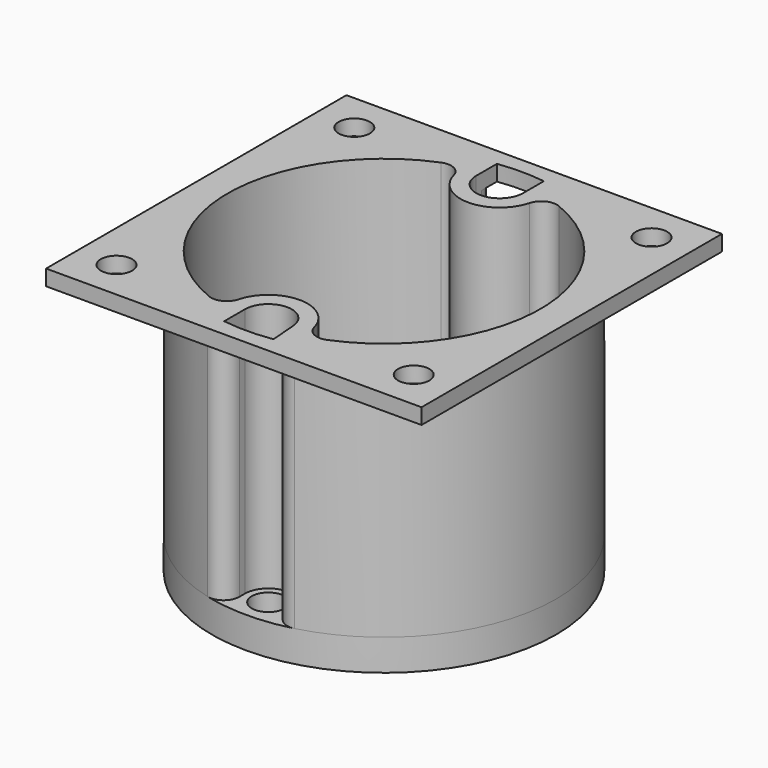
from build123d import *

# Parameters (mm, degrees)
F0_R         = 34.925
F1_DEPTH     = 6.35
F3_DEPTH     = 50.8
F4_R         = 3.3655
F5_DEPTH     = 6.35
F6_W         = 76.2
F6_H         = 76.2
F6_R         = 34.925
F7_DEPTH     = 3.175
F8_R         = 3.175
F9_DEPTH     = 3.175
F10_T1_DEPTH = 50.8
F10_T3_DEPTH = 47.625
F12_DEPTH    = 6.35
F13_R        = 3.175


# Not quite as in the source:
# - a fillet or chamfer that OpenCascade refuses, or shapes differently, is made with other operations: its cross-section is extruded or revolved along the edge and cut away or added


with BuildPart() as f1:
    # F0 (on Top) → F1 (new body)
    with BuildSketch(Plane.XY):
        Circle(F0_R)
    extrude(amount=F1_DEPTH)

    # F2 (on face) → F3 (join)
    with BuildSketch(Plane.XY.offset(6.35)):
        with BuildLine():
            ThreePointArc((4.7625, 29.337), (0, 24.5745), (-4.7625, 29.337))
            Line((-4.7625, 29.337), (-4.7625, 34.5987603644))
            ThreePointArc((-4.7625, 34.5987603644), (-34.925, 0), (-4.7625, -34.5987603644))
            Line((-4.7625, -34.5987603644), (-4.7625, -29.337))
            ThreePointArc((-4.7625, -29.337), (-0.1934429178, -24.5784302477), (4.7467854961, -28.9504334416))
            Line((4.7467854961, -28.9504334416), (5.2016172982, -34.5354716557))
            ThreePointArc((5.2016172982, -34.5354716557), (26.4709473682, -22.7825496912), (34.925, 0))
            ThreePointArc((34.925, 0), (26.3257092734, 22.950221268), (4.7625, 34.5987603644))
            Line((4.7625, 34.5987603644), (4.7625, 29.337))
        make_face()
        with BuildLine():
            ThreePointArc((-7.9375, -30.7418053105), (-31.75, 0), (-7.9375, 30.7418053105))
            Line((-7.9375, 30.7418053105), (-7.9375, 29.337))
            ThreePointArc((-7.9375, 29.337), (0, 21.3995), (7.9375, 29.337))
            Line((7.9375, 29.337), (7.9375, 30.7418053105))
            ThreePointArc((7.9375, 30.7418053105), (31.7499202127, 0.0711792809), (8.075257951, -30.7059067449))
            Line((8.075257951, -30.7059067449), (7.9113091602, -28.6927224026))
            ThreePointArc((7.9113091602, -28.6927224026), (-0.3224048629, -21.4060504128), (-7.9375, -29.337))
            Line((-7.9375, -29.337), (-7.9375, -30.7418053105))
        make_face(mode=Mode.SUBTRACT)
    extrude(amount=F3_DEPTH)

    # F4 (on face) → F5 (cut, through all)
    with BuildSketch(Plane.XY.offset(6.35)):
        with Locations((0, 29.337)):
            Circle(F4_R)
        with Locations((0, -29.337)):
            Circle(F4_R)
    extrude(amount=-F5_DEPTH, mode=Mode.SUBTRACT)

    # F6 (on face) → F7 (join)
    with BuildSketch(Plane.XY.offset(57.15)):
        Rectangle(F6_W, F6_H)
        Circle(F6_R, mode=Mode.SUBTRACT)
    extrude(amount=-F7_DEPTH)

    # F8 (on face) → F9 (cut, through all)
    with BuildSketch(Plane.XY.offset(57.15)):
        with Locations((-30.1625, 30.1625)):
            Circle(F8_R)
        with Locations((30.1625, 30.1625)):
            Circle(F8_R)
        with Locations((-30.1625, -30.1625)):
            Circle(F8_R)
        with Locations((30.1625, -30.1625)):
            Circle(F8_R)
    extrude(amount=-F9_DEPTH, mode=Mode.SUBTRACT)

    # F10: fillet of radius 3.175 on 8 edges, made by hand

    # F10_s2 → F10_t1 (join)
    with BuildSketch(Plane.XY.offset(6.35)):
        with BuildLine():
            ThreePointArc((-7.6707325335, -27.2964685374), (-9.3216408312, -29.3213201135), (-11.9322506076, -29.4225066138))
            Line((-11.9322506076, -29.4225066138), (-12.0515731137, -29.7167316799))
            ThreePointArc((-12.0515731137, -29.7167316799), (-10.0563182102, -30.4498771805), (-8.016875, -31.0492233636))
            Line((-8.016875, -31.0492233636), (-7.62, -30.7418053105))
            ThreePointArc((-7.62, -30.7418053105), (-7.62, -29.337), (-7.3639032321, -27.3780897959))
            Line((-7.3639032321, -27.3780897959), (-7.6707325335, -27.2964685374))
        make_face()
        with BuildLine():
            ThreePointArc((7.6707325335, -27.2964685374), (9.3216408312, -29.3213201135), (11.9322506076, -29.4225066138))
            Line((11.9322506076, -29.4225066138), (12.0515731137, -29.7167316799))
            ThreePointArc((12.0515731137, -29.7167316799), (10.1245575171, -30.4272557312), (8.1560105306, -31.0129658123))
            Line((8.1560105306, -31.0129658123), (7.7588055846, -30.7316778488))
            ThreePointArc((7.7588055846, -30.7316778488), (7.5948567937, -28.7184935065), (7.3639032321, -27.3780897959))
            Line((7.3639032321, -27.3780897959), (7.6707325335, -27.2964685374))
        make_face()
        with BuildLine():
            ThreePointArc((-11.9322506076, 29.4225066138), (-9.3216408312, 29.3213201135), (-7.6707325335, 27.2964685374))
            Line((-7.6707325335, 27.2964685374), (-7.3639032321, 27.3780897959))
            ThreePointArc((-7.3639032321, 27.3780897959), (-7.62, 29.337), (-7.62, 30.7418053105))
            Line((-7.62, 30.7418053105), (-8.016875, 31.0492233636))
            ThreePointArc((-8.016875, 31.0492233636), (-10.0563182102, 30.4498771805), (-12.0515731137, 29.7167316799))
            Line((-12.0515731137, 29.7167316799), (-11.9322506076, 29.4225066138))
        make_face()
        with BuildLine():
            ThreePointArc((11.9322506076, 29.4225066138), (9.3216408312, 29.3213201135), (7.6707325335, 27.2964685374))
            Line((7.6707325335, 27.2964685374), (7.3639032321, 27.3780897959))
            ThreePointArc((7.3639032321, 27.3780897959), (7.62, 29.337), (7.62, 30.7418053105))
            Line((7.62, 30.7418053105), (8.016875, 31.0492233636))
            ThreePointArc((8.016875, 31.0492233636), (10.0563182102, 30.4498771805), (12.0515731137, 29.7167316799))
            Line((12.0515731137, 29.7167316799), (11.9322506076, 29.4225066138))
        make_face()
    extrude(amount=F10_T1_DEPTH)

    # F10_s4 → F10_t3 (cut)
    with BuildSketch(Plane.XY.offset(6.35)):
        with BuildLine():
            ThreePointArc((-8.73125, -33.8159858416), (-5.9932175167, -33.2518632033), (-4.7625, -30.7418053105))
            Line((-4.7625, -30.7418053105), (-4.7625, -34.5987603644))
            ThreePointArc((-4.7625, -34.5987603644), (-6.7582176832, -34.2648817121), (-8.73125, -33.8159858416))
        make_face()
        with BuildLine():
            ThreePointArc((8.8827837461, -33.7764974193), (6.2403375987, -33.2969861146), (4.910734287, -30.9636177838))
            Line((4.910734287, -30.9636177838), (5.2016172982, -34.5354716557))
            ThreePointArc((5.2016172982, -34.5354716557), (7.0524179305, -34.2055408718), (8.8827837461, -33.7764974193))
        make_face()
        with BuildLine():
            ThreePointArc((8.73125, 33.8159858416), (5.9932175167, 33.2518632033), (4.7625, 30.7418053105))
            Line((4.7625, 30.7418053105), (4.7625, 34.5987603644))
            ThreePointArc((4.7625, 34.5987603644), (6.7582176832, 34.2648817121), (8.73125, 33.8159858416))
        make_face()
        with BuildLine():
            ThreePointArc((-8.73125, 33.8159858416), (-5.9932175167, 33.2518632033), (-4.7625, 30.7418053105))
            Line((-4.7625, 30.7418053105), (-4.7625, 34.5987603644))
            ThreePointArc((-4.7625, 34.5987603644), (-6.7582176832, 34.2648817121), (-8.73125, 33.8159858416))
        make_face()
    extrude(amount=F10_T3_DEPTH, mode=Mode.SUBTRACT)

    # F11 (on Top) → F12 (cut, through all)
    with BuildSketch(Plane.XY):
        with BuildLine():
            ThreePointArc((7.7858076955, 27.4938506494), (0, 21.336), (-7.7858076955, 27.4938506494))
            ThreePointArc((-7.7858076955, 27.4938506494), (-28.575, 0), (-7.7858076955, -27.4938506494))
            ThreePointArc((-7.7858076955, -27.4938506494), (0, -21.336), (7.7858076955, -27.4938506494))
            ThreePointArc((7.7858076955, -27.4938506494), (28.575, 0), (7.7858076955, 27.4938506494))
        make_face()
    extrude(amount=F12_DEPTH, mode=Mode.SUBTRACT)

    # F13
    f13_edges = [f1.edges().sort_by_distance(p)[0] for p in [
        (-7.785808, 27.493851, 3.175),
        (7.785808, 27.493851, 3.175),
        (-7.785808, -27.493851, 3.175),
        (7.785808, -27.493851, 3.175),
    ]]
    fillet(f13_edges, radius=F13_R)


solid = f1.part
